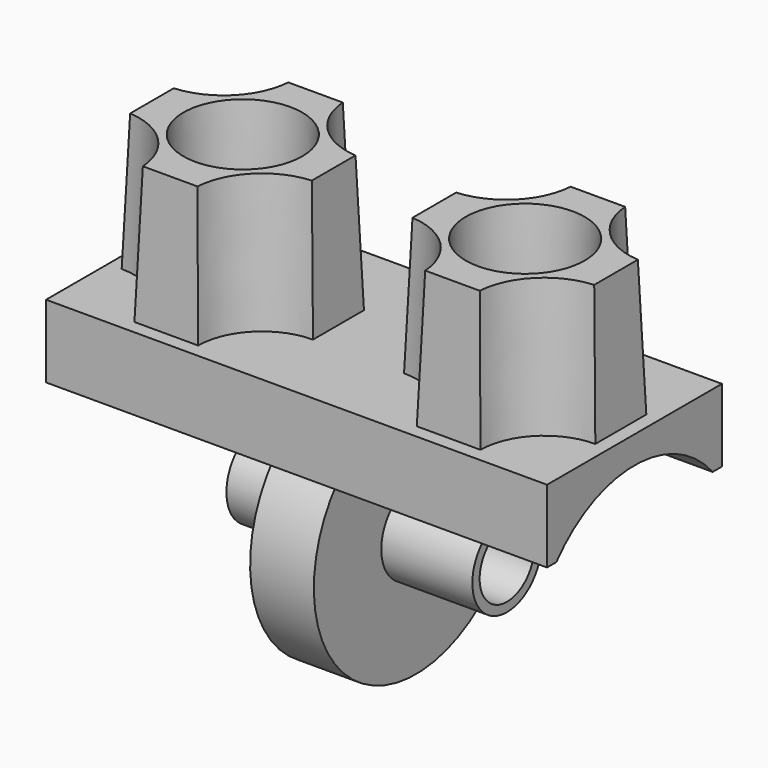
from build123d import *

# Parameters (mm, degrees)
F0_W                    = 550
F0_H                    = 240
F1_DEPTH                = 80
F3_DEPTH                = 656.54541
F4_R                    = 140
F5_DEPTH                = 35
F5_DEPTH_BACK           = 35
F6_R                    = 47.5
F6_R_2                  = 37.5
F7_DEPTH                = 100
F9_R                    = 60
F10_DEPTH               = 150
DRAFT_F10_DRAFTED_ANGLE = 2


# Not quite as in the source:
# - an extrude with a draft is written as a straight extrude whose walls are then drafted


with BuildPart() as f1:
    # F0 (on Top) → F1 (new body)
    with BuildSketch(Plane.XY):
        Rectangle(F0_W, F0_H)
    extrude(amount=F1_DEPTH)

    # F2 (on face) → F3 (cut)
    with BuildSketch(Plane(origin=(-275, 0, 0), x_dir=(0, -1, 0), z_dir=(-1, 0, 0))):
        with BuildLine():
            ThreePointArc((-107.2380529476, 0), (-47.8887908979, -221.5547935513), (140, -90))
            ThreePointArc((140, -90), (131.5547935513, -42.1112091021), (107.2380529476, 0))
            Line((107.2380529476, 0), (-107.2380529476, 0))
        make_face()
        with BuildLine():
            Line((-107.2380529476, 0), (107.2380529476, 0))
            ThreePointArc((107.2380529476, 0), (0, 50), (-107.2380529476, 0))
        make_face()
    extrude(amount=-F3_DEPTH, mode=Mode.SUBTRACT)

    # F4 (on Right) → F5 (join, two sides)
    with BuildSketch(Plane.YZ) as f5_sk:
        with Locations((0, -90)):
            Circle(F4_R)
    extrude(amount=F5_DEPTH)
    extrude(f5_sk.sketch, amount=-F5_DEPTH_BACK)

    # F6 (on face) → F7 (join)
    with BuildSketch(Plane.YZ.offset(35)):
        with Locations((0, -90)):
            Circle(F6_R)
        with Locations((0, -90)):
            Circle(F6_R_2, mode=Mode.SUBTRACT)
    extrude(amount=F7_DEPTH)

    # F8: F1 across plane


with BuildPart() as f1_1:
    add(f1.part)
    add(f1.part.mirror(Plane.YZ))


with BuildPart() as f10_drafted:
    # F9 (on face) → F10 (new body)
    with BuildSketch(Plane.XY.offset(80)):
        with BuildLine():
            Line((-190, -105), (-120, -105))
            ThreePointArc((-120, -105), (-99.4974746831, -55.5025253169), (-50, -35))
            Line((-50, -35), (-50, 35))
            ThreePointArc((-50, 35), (-99.4974746831, 55.5025253169), (-120, 105))
            Line((-120, 105), (-190, 105))
            ThreePointArc((-190, 105), (-210.5025253169, 55.5025253169), (-260, 35))
            Line((-260, 35), (-260, -35))
            ThreePointArc((-260, -35), (-210.5025253169, -55.5025253169), (-190, -105))
        make_face()
        with Locations((-155, 0)):
            Circle(F9_R, mode=Mode.SUBTRACT)
    extrude(amount=F10_DEPTH)

    # draft_F10_drafted
    draft_f10_drafted_walls = [f10_drafted.faces().sort_by_distance(p)[0] for p in [
        (-155, -105, 180),
        (-99.4974746831, -55.5025253169, 180),
        (-50, 0, 180),
        (-99.4974746831, 55.5025253169, 180),
        (-155, 105, 180),
        (-210.5025253169, 55.5025253169, 180),
        (-260, 0, 180),
        (-210.5025253169, -55.5025253169, 180),
        (-215, 0, 180),
    ]]
    draft(draft_f10_drafted_walls, neutral_plane=Plane.XY.offset(80), angle=DRAFT_F10_DRAFTED_ANGLE)


with BuildPart() as f1_2:
    add(f1_1.part)

    # join_F10_drafted: union F10_drafted
    add(f10_drafted.part)

    # F11: F1 across plane


with BuildPart() as f1_3:
    add(f1_2.part)
    add(f1_2.part.mirror(Plane.YZ))


solid = f1_3.part
